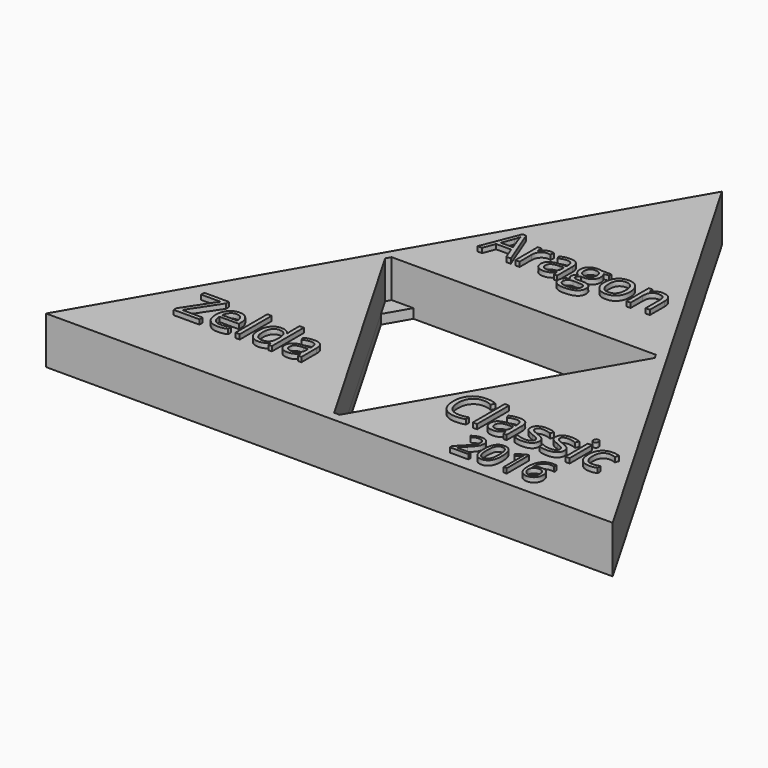
from build123d import *

# Parameters (mm, degrees)
F1_DEPTH       = 5
F3_DEPTH       = 4
F5_DEPTH       = 25
F6_TEXT_SIZE   = 5.5555555556
F6_TEXT_SIZE_2 = 4.1666666667
F7_DEPTH       = 0.5


# Not quite as in the source:
# - Text() gives the source's letters only with a copy of the font that has no kerning and outlines rounded to 1/6400 em; it was checked with that copy


with BuildPart() as f1:
    # F0 (on Top) → F1 (new body)
    with BuildSketch(Plane.XY):
        Polygon((0, 30), (-30, -21.9615242271), (30, -21.9615242271), align=None)
    extrude(amount=F1_DEPTH)

    # F2 (on face) → F3 (cut)
    with BuildSketch(Plane.XY.offset(5)):
        Polygon((-13.9896370289, 3.7692378865), (-14.2783121635, 3.2692378865), (-0.2886751346, -20.9615242271), (0.2886751346, -20.9615242271), (14.2783121635, 3.2692378865), (13.9896370289, 3.7692378865), align=None)
    extrude(amount=-F3_DEPTH, mode=Mode.SUBTRACT)

    # F4 (on face) → F5 (cut)
    with BuildSketch(Plane.XY.offset(1)):
        Polygon((13.1236116251, 1.2692378865), (11.6802359522, 3.7692378865), (-11.6802359522, 3.7692378865), (-13.1236116251, 1.2692378865), (-1.443375673, -18.9615242271), (1.443375673, -18.9615242271), align=None)
    extrude(amount=-F5_DEPTH, mode=Mode.SUBTRACT)

    # F6 (on face) → F7 (join)
    with BuildSketch(Plane.XY.offset(5)):
        with Locations((-9.0671446262, 8.9965035289)):
            Text('Aragon', F6_TEXT_SIZE, font='Open Sans', text_align=(TextAlign.LEFT, TextAlign.BOTTOM))
        with Locations((-21.7939833034, -15.6044296764)):
            Text('Zelda', F6_TEXT_SIZE, font='Open Sans', text_align=(TextAlign.LEFT, TextAlign.BOTTOM))
        with Locations((6.3589551413, -15.8943415393)):
            Text('Classic', F6_TEXT_SIZE, font='Open Sans', text_align=(TextAlign.LEFT, TextAlign.BOTTOM))
        with Locations((11.4357401467, -20.5585775374)):
            Text('2016', F6_TEXT_SIZE_2, font='Open Sans', text_align=(TextAlign.LEFT, TextAlign.BOTTOM))
    extrude(amount=F7_DEPTH)


solid = f1.part
